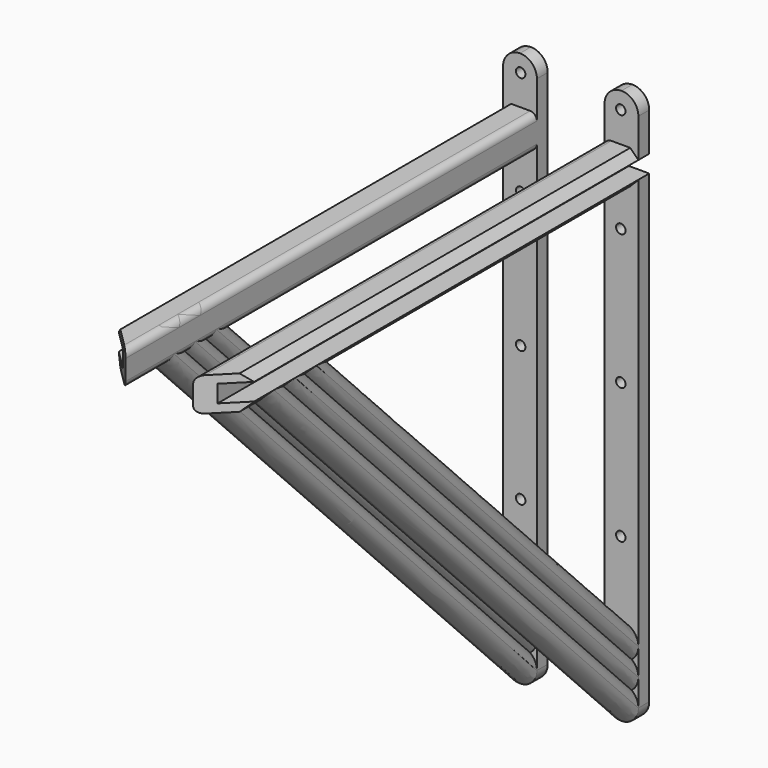
from build123d import *

# Parameters (mm, degrees)
F0_W        = 96.52
F0_H        = 6.35
F1_DEPTH    = 2.54
F2_W        = 96.52
F2_H        = 1.524
F2_H_2      = 1.5748
F3_DEPTH    = 3.81
F5_DEPTH    = 6.351
F6_T1_DEPTH = 98.0084897473
F7_R        = 1.27
F9_DEPTH    = 2.54
F15_DEPTH   = 25.4
F16_R       = 0.889
F17_DEPTH   = 25.4
F18_R       = 3.1749


# Not quite as in the source:
# - a fillet or chamfer that OpenCascade refuses, or shapes differently, is made with other operations: its cross-section is extruded or revolved along the edge and cut away or added
# - a fillet or chamfer is up to 0.001 mm smaller than in the source, because OpenCascade refuses the exact size


with BuildPart() as f1:
    # F0 (on Right) → F1 (new body)
    with BuildSketch(Plane.YZ):
        with Locations((42.4467639691, 3.1188557479)):
            Rectangle(F0_W, F0_H)
    extrude(amount=F1_DEPTH)

    # F2 (on face) → F3 (join)
    with BuildSketch(Plane.YZ.offset(2.54)):
        with Locations((42.4467639691, 5.5318557479)):
            Rectangle(F2_W, F2_H)
        with Locations((42.4467639691, 0.7312557479)):
            Rectangle(F2_W, F2_H_2)
    extrude(amount=F3_DEPTH)

    # F4 (on face) → F5 (cut, through all)
    with BuildSketch(Plane.XY.offset(6.2938557479)):
        Polygon((12.7, 6.8867639691), (0, -5.8132360309), (12.7, -5.8132360309), align=None)
    extrude(amount=-F5_DEPTH, mode=Mode.SUBTRACT)

    # F6: chamfer of 1.524 on 2 edges, made by hand

    # F6_s2 → F6_t1 (cut)
    with BuildSketch(Plane.XZ.offset(-94.6260088427)):
        Polygon((6.35, 4.7698557479), (4.826, 6.2938557479), (6.35, 6.2938557479), align=None)
        Polygon((4.826, -0.0561442521), (6.35, 1.4678557479), (6.35, -0.0561442521), align=None)
    extrude(amount=F6_T1_DEPTH, mode=Mode.SUBTRACT)

    # F7
    f7_edges = [f1.edges().sort_by_distance(p)[0] for p in [
        (0, 42.446764, 6.293856),
        (0, 42.446764, -0.056144),
    ]]
    fillet(f7_edges, radius=F7_R)

    # F8 (on face) → F9 (join)
    with BuildSketch(Plane(origin=(0, 90.7067639691, 0), x_dir=(-1, 0, 0), z_dir=(0, 1, 0))):
        with BuildLine():
            Line((0, -88.9561442521), (0, 1.2138557479))
            ThreePointArc((0, 1.2138557479), (-0.3719743879, 0.3158301358), (-1.27, -0.0561442521))
            Line((-1.27, -0.0561442521), (-4.826, -0.0561442521))
            Line((-4.826, -0.0561442521), (-6.35, 1.4678557479))
            Line((-6.35, 1.4678557479), (-6.35, -88.9561442521))
            Line((-6.35, -88.9561442521), (0, -88.9561442521))
        make_face()
        with BuildLine():
            Line((0, 5.0238557479), (0, 15.1838557479))
            Line((0, 15.1838557479), (-6.35, 15.1838557479))
            Line((-6.35, 15.1838557479), (-6.35, 4.7698557479))
            Line((-6.35, 4.7698557479), (-4.826, 6.2938557479))
            Line((-4.826, 6.2938557479), (-1.27, 6.2938557479))
            ThreePointArc((-1.27, 6.2938557479), (-0.3719743879, 5.92188136), (0, 5.0238557479))
        make_face()
        with BuildLine():
            Line((0, 1.2138557479), (0, 5.0238557479))
            ThreePointArc((0, 5.0238557479), (-0.3719743879, 5.92188136), (-1.27, 6.2938557479))
            Line((-1.27, 6.2938557479), (-4.826, 6.2938557479))
            Line((-4.826, 6.2938557479), (-6.35, 4.7698557479))
            Line((-6.35, 4.7698557479), (-2.54, 4.7698557479))
            Line((-2.54, 4.7698557479), (-2.54, 1.5186557479))
            Line((-2.54, 1.5186557479), (-6.35, 1.5186557479))
            Line((-6.35, 1.5186557479), (-6.35, 1.4678557479))
            Line((-6.35, 1.4678557479), (-4.826, -0.0561442521))
            Line((-4.826, -0.0561442521), (-1.27, -0.0561442521))
            ThreePointArc((-1.27, -0.0561442521), (-0.3719743879, 0.3158301358), (0, 1.2138557479))
        make_face()
    extrude(amount=F9_DEPTH)

    # F13: sweep along a path in F12
    with BuildLine(Plane.YZ.offset(3.175)) as f13_path:
        Line((90.7067639691, -88.9561442521), (3.5845157613, 0))
    # F10 (on face) → F13 (sweep)
    with BuildSketch(Plane.XZ.offset(-90.7067639691)):
        with BuildLine():
            ThreePointArc((0, -80.7011442521), (0.3351936686, -82.1210474178), (1.27, -83.2411442521))
            ThreePointArc((1.27, -83.2411442521), (0.3351936652, -84.3612410931), (0, -85.7811442672))
            ThreePointArc((0, -85.7811442672), (0.929935975, -88.0262082877), (3.175, -88.9561442521))
            ThreePointArc((3.175, -88.9561442521), (5.4200640303, -88.0262082824), (6.35, -85.7811442521))
            ThreePointArc((6.35, -85.7811442521), (6.0148063314, -84.3612410864), (5.08, -83.2411442521))
            ThreePointArc((5.08, -83.2411442521), (6.0148063314, -82.1210474178), (6.35, -80.7011442521))
            ThreePointArc((6.35, -80.7011442521), (6.0148063314, -79.2812410864), (5.08, -78.1611442521))
            ThreePointArc((5.08, -78.1611442521), (6.0148063348, -77.0410474111), (6.35, -75.6211442371))
            ThreePointArc((6.35, -75.6211442371), (3.1749999925, -72.4461442521), (0, -75.6211442521))
            ThreePointArc((0, -75.6211442521), (0.3351936686, -77.0410474178), (1.27, -78.1611442521))
            ThreePointArc((1.27, -78.1611442521), (0.3351936686, -79.2812410864), (0, -80.7011442521))
        make_face()
    sweep(path=f13_path.line)

    # F14 (on face) → F15 (cut)
    with BuildSketch(Plane.XZ.offset(-3.5845157613)):
        Polygon((8.343354216, 2.9688845389), (6.35, 4.7698557479), (2.54, 4.7698557479), (2.54, 1.5186557479), (6.35, 1.5186557479), align=None)
        with BuildLine():
            Line((4.826, 6.2938557479), (6.35, 4.7698557479))
            Line((6.35, 4.7698557479), (9.041506215, 18.2706966987))
            Line((9.041506215, 18.2706966987), (0, 17.7238557479))
            Line((0, 17.7238557479), (0, 5.0238557479))
            ThreePointArc((0, 5.0238557479), (0.3719743879, 5.92188136), (1.27, 6.2938557479))
            Line((1.27, 6.2938557479), (4.826, 6.2938557479))
        make_face()
    extrude(amount=-F15_DEPTH, mode=Mode.SUBTRACT)

    # F16 (on face) → F17 (cut)
    with BuildSketch(Plane.XZ.offset(-90.7067639691)):
        with Locations((3.048, 12.0088557479)):
            Circle(F16_R)
        with Locations((3.048, -7.6761442521)):
            Circle(F16_R)
        with Locations((3.048, -33.0761442521)):
            Circle(F16_R)
        with Locations((3.048, -58.4761442521)):
            Circle(F16_R)
    extrude(amount=-F17_DEPTH, mode=Mode.SUBTRACT)

    # F18 (radius 3.175 in the source; OpenCascade refuses exactly that, so slightly less here)
    f18_edges = [f1.edges().sort_by_distance(p)[0] for p in [
        (6.35, 91.976764, 15.183856),
        (0, 91.976764, 15.183856),
        (6.35, 91.976764, -88.956144),
        (0, 91.976764, -88.956144),
    ]]
    fillet(f18_edges, radius=F18_R)


with BuildPart() as f20_1:
    # F20: instance of F1
    add(f1.part.mirror(Plane.YZ.offset(-6.35)))


solid = Compound([f1.part, f20_1.part])
